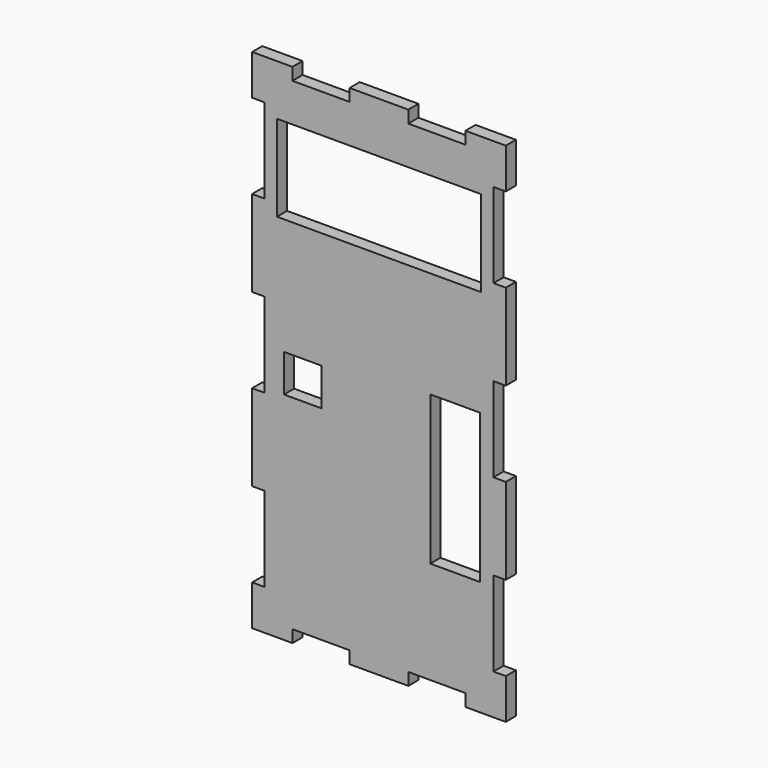
from build123d import *

# Parameters (mm, degrees)
F0_W     = 63.5
F0_H     = 127
F0_W_2   = 9.398
F0_H_2   = 9.398
F0_W_3   = 12.4
F0_H_3   = 37.3
F0_W_4   = 51.054
F0_H_4   = 21.59
F1_DEPTH = 3.175
F2_W     = 14.3
F2_H     = 3.075
F2_W_2   = 3.075
F2_H_2   = 21.2
F3_DEPTH = 25


# Not quite as in the source:
# - a feature of the source that left no trace in its solid (it failed there, or was rolled back) is left out
# - a length typed as a fraction of an inch, garbled in the dataset ("3 / 203.2 mm" for 3/8 in), is restored


with BuildPart() as f1:
    # F0 (on Front) → F1 (new body)
    with BuildSketch(Plane.XZ):
        Rectangle(F0_W, F0_H)
        with Locations((-19.05, -4.699)):
            Rectangle(F0_W_2, F0_H_2, mode=Mode.SUBTRACT)
        with Locations((19.05, -16.11)):
            Rectangle(F0_W_3, F0_H_3, mode=Mode.SUBTRACT)
        with Locations((0, 40.005)):
            Rectangle(F0_W_4, F0_H_4, mode=Mode.SUBTRACT)
    extrude(amount=-F1_DEPTH)

    # F2 (on face) → F3 (cut)
    with BuildSketch(Plane(origin=(0, 3.175, 0), x_dir=(-1, 0, 0), z_dir=(0, 1, 0))):
        with Locations((14.5, 61.9625)):
            Rectangle(F2_W, F2_H)
        with Locations((-14.5, 61.9625)):
            Rectangle(F2_W, F2_H)
        with Locations((-30.2125, -42.8)):
            Rectangle(F2_W_2, F2_H_2)
        with Locations((-30.2125, 0)):
            Rectangle(F2_W_2, F2_H_2)
        with Locations((-30.2125, 42.8)):
            Rectangle(F2_W_2, F2_H_2)
        with Locations((30.2125, -42.8)):
            Rectangle(F2_W_2, F2_H_2)
        with Locations((30.2125, 0)):
            Rectangle(F2_W_2, F2_H_2)
        with Locations((30.2125, 42.8)):
            Rectangle(F2_W_2, F2_H_2)
        with Locations((-14.5, -61.9625)):
            Rectangle(F2_W, F2_H)
        with Locations((14.5, -61.9625)):
            Rectangle(F2_W, F2_H)
    extrude(amount=-F3_DEPTH, mode=Mode.SUBTRACT)


solid = f1.part
